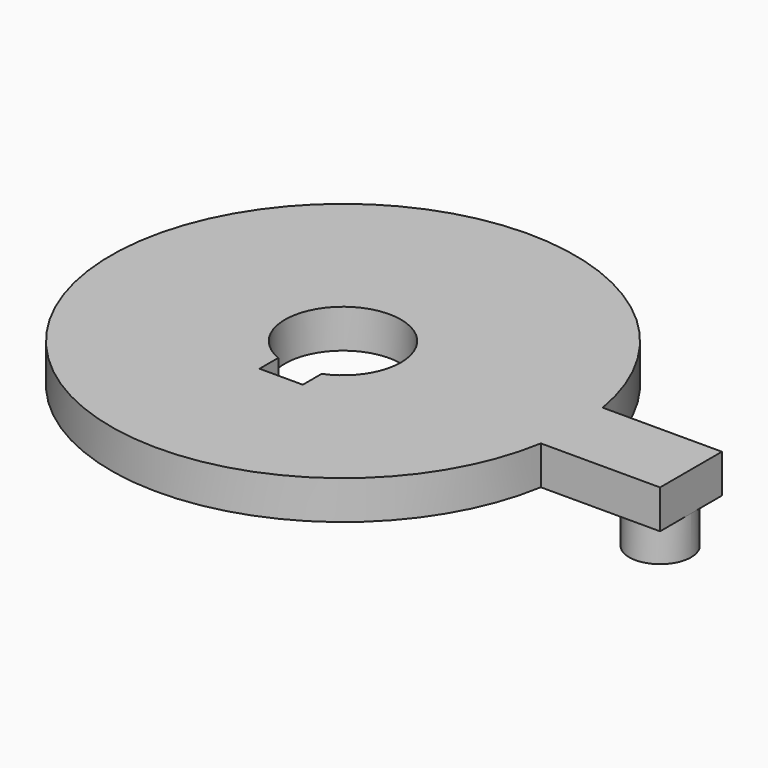
from build123d import *

# Parameters (mm, degrees)
F1_DEPTH = 2.5
F2_R     = 4
F3_DEPTH = 5


with BuildPart() as f1:
    # F0 (on Top) → F1 (new body, symmetric)
    with BuildSketch(Plane.XY):
        with BuildLine():
            ThreePointArc((29.5803989155, -5), (29.8949156836, -2.5087878084), (30, 0))
            ThreePointArc((30, 0), (29.8949156836, 2.5087878084), (29.5803989155, 5))
            ThreePointArc((29.5803989155, 5), (-30, 0), (29.5803989155, -5))
        make_face()
        with BuildLine():
            ThreePointArc((-2.8, -6.9577295147), (-4.1982139059, 6.2149014473), (7.5, 0))
            ThreePointArc((7.5, 0), (6.2149014473, -4.1982139059), (2.8, -6.9577295147))
            Line((2.8, -6.9577295147), (2.8, -10))
            Line((2.8, -10), (0, -10))
            Line((0, -10), (-2.8, -10))
            Line((-2.8, -10), (-2.8, -6.9577295147))
        make_face(mode=Mode.SUBTRACT)
        with BuildLine():
            ThreePointArc((29.5803989155, 5), (29.8949156836, 2.5087878084), (30, 0))
            ThreePointArc((30, 0), (29.8949156836, -2.5087878084), (29.5803989155, -5))
            Line((29.5803989155, -5), (45, -5))
            Line((45, -5), (45, 0))
            Line((45, 0), (45, 5))
            Line((45, 5), (29.5803989155, 5))
        make_face()
    extrude(amount=F1_DEPTH, both=True)

    # F2 (on face) → F3 (join)
    with BuildSketch(Plane(origin=(0, 0, -2.5), x_dir=(1, 0, 0), z_dir=(0, 0, -1))):
        with Locations((41.0000477707, -0.0195490011)):
            Circle(F2_R)
    extrude(amount=F3_DEPTH)


solid = f1.part
